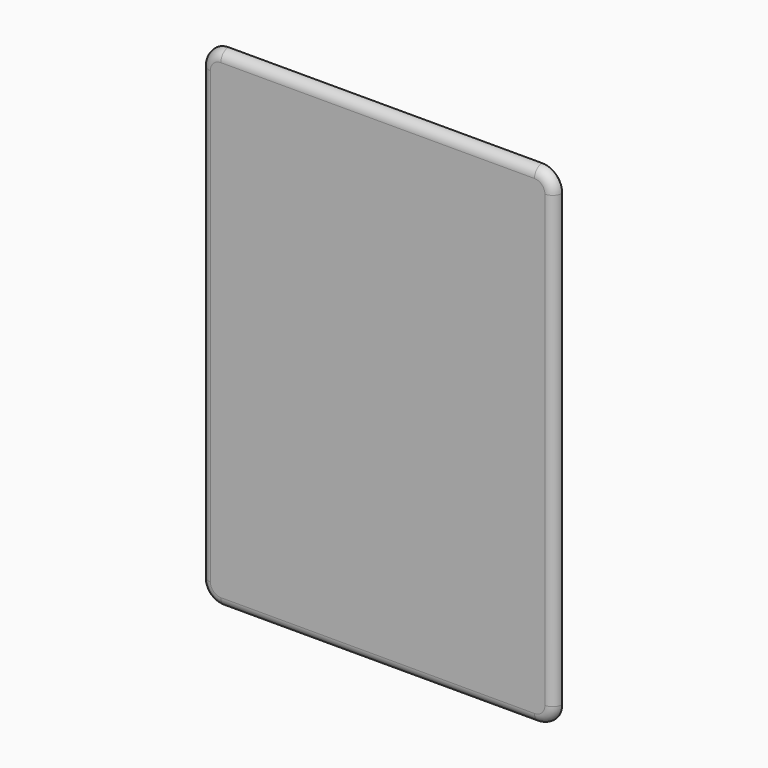
from build123d import *

# Parameters (mm, degrees)
F1_DEPTH = 6.9
F2_R     = 6
F3_SIZE  = 0.89999


# Not quite as in the source:
# - a fillet or chamfer is up to 0.001 mm smaller than in the source, because OpenCascade refuses the exact size


with BuildPart() as f1:
    # F0 (on Front) → F1 (new body)
    with BuildSketch(Plane.XZ):
        with BuildLine():
            Line((97.8, 152.85), (-97.8, 152.85))
            ThreePointArc((-97.8, 152.85), (-106.6388347648, 149.1888347648), (-110.3, 140.35))
            Line((-110.3, 140.35), (-110.3, -140.35))
            ThreePointArc((-110.3, -140.35), (-106.6388347648, -149.1888347648), (-97.8, -152.85))
            Line((-97.8, -152.85), (97.8, -152.85))
            ThreePointArc((97.8, -152.85), (106.6388347648, -149.1888347648), (110.3, -140.35))
            Line((110.3, -140.35), (110.3, 140.35))
            ThreePointArc((110.3, 140.35), (106.6388347648, 149.1888347648), (97.8, 152.85))
        make_face()
    extrude(amount=F1_DEPTH)

    # F2
    f2_edges = [f1.edges().sort_by_distance(p)[0] for p in [
        (110.3, -6.9, 0),
        (106.638835, -6.9, 149.188835),
        (0, -6.9, 152.85),
        (-106.638835, -6.9, 149.188835),
        (-110.3, -6.9, 0),
        (-106.638835, -6.9, -149.188835),
        (0, -6.9, -152.85),
        (106.638835, -6.9, -149.188835),
    ]]
    fillet(f2_edges, radius=F2_R)

    # F3 (size 0.9 in the source; OpenCascade refuses exactly that, so slightly less here)
    f3_edges = [f1.edges().sort_by_distance(p)[0] for p in [
        (110.3, 0, 0),
        (106.638835, 0, 149.188835),
        (0, 0, 152.85),
        (-106.638835, 0, 149.188835),
        (-110.3, 0, 0),
        (-106.638835, 0, -149.188835),
        (0, 0, -152.85),
        (106.638835, 0, -149.188835),
    ]]
    chamfer(f3_edges, length=F3_SIZE)


solid = f1.part
